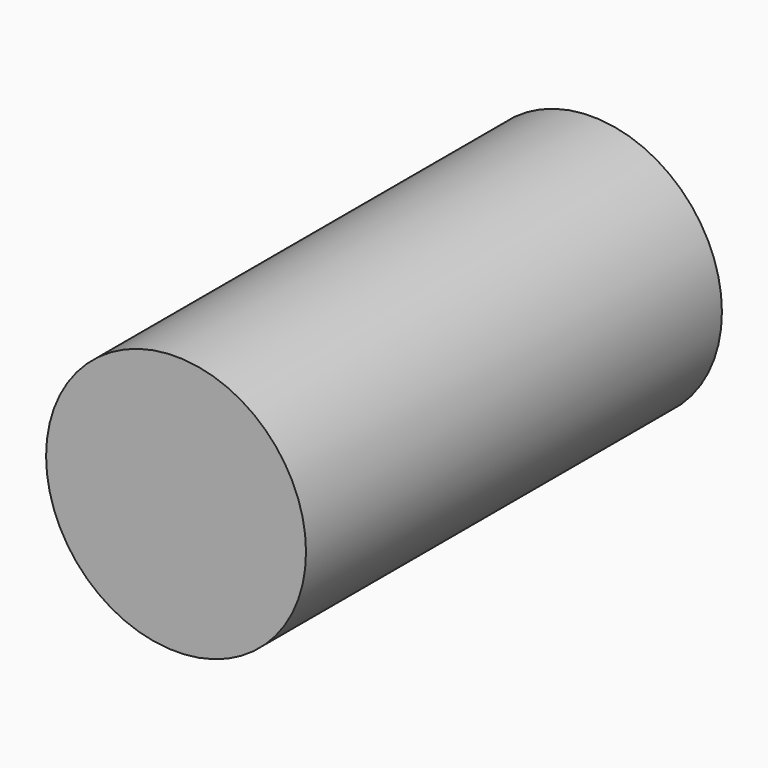
from build123d import *

# Parameters (mm, degrees)
F0_R     = 25
F1_DEPTH = 100


# Not quite as in the source:
# - the program builds the solid bodies; features that only make, move or delete a surface that nothing else refers to are left out


with BuildPart() as f1:
    # F0 (on Front) → F1 (new body)
    with BuildSketch(Plane.XZ):
        Circle(F0_R)
    extrude(amount=F1_DEPTH)


solid = f1.part
